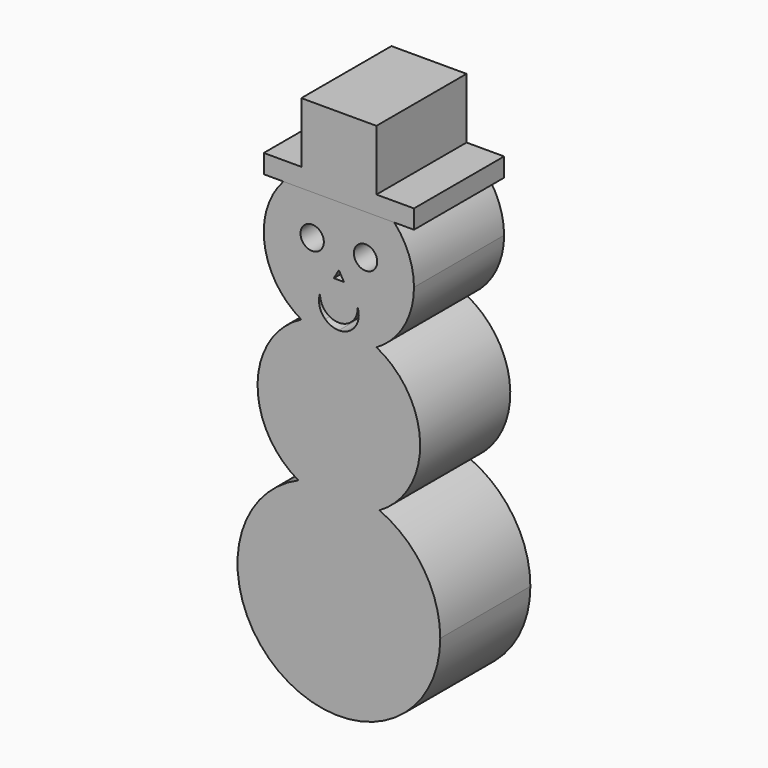
from build123d import *

# Parameters (mm, degrees)
F0_R     = 3.9452510547
F1_DEPTH = 38.1
F2_W     = 12.7
F2_H     = 20.4561264838
F3_DEPTH = 38.1
F4_DEPTH = 38.1


with BuildPart() as f1:
    # F0 (on Front) → F1 (new body)
    with BuildSketch(Plane.XZ):
        with BuildLine():
            ThreePointArc((13.7157117337, -23.8302700758), (23.8025510421, -13.7637598111), (27.4955, 0))
            ThreePointArc((27.4955, 0), (23.5116729393, 14.2549554838), (12.714626341, 24.3791057518))
            ThreePointArc((12.714626341, 24.3791057518), (0, 20.9677), (-12.714626341, 24.3791057518))
            ThreePointArc((-12.714626341, 24.3791057518), (-27.4895738801, 0.5708310965), (-13.7157117337, -23.8302700758))
            ThreePointArc((-13.7157117337, -23.8302700758), (0, -20.9677), (13.7157117337, -23.8302700758))
        make_face()
        with BuildLine():
            ThreePointArc((-12.714626341, 24.3791057518), (0, 20.9677), (12.714626341, 24.3791057518))
            ThreePointArc((12.714626341, 24.3791057518), (8.7732416217, 26.0582568814), (4.6188620822, 27.1047714123))
            ThreePointArc((4.6188620822, 27.1047714123), (2.4852773653, 25.7442761783), (0, 25.2683271861))
            ThreePointArc((0, 25.2683271861), (-2.4852773653, 25.7442761783), (-4.6188620822, 27.1047714123))
            ThreePointArc((-4.6188620822, 27.1047714123), (-8.7732416217, 26.0582568814), (-12.714626341, 24.3791057518))
        make_face()
        with BuildLine():
            ThreePointArc((4.6188620822, 27.1047714123), (8.7732416217, 26.0582568814), (12.714626341, 24.3791057518))
            ThreePointArc((12.714626341, 24.3791057518), (22.0012671119, 33.6750152773), (25.4, 46.3677))
            ThreePointArc((25.4, 46.3677), (-12.6926847227, 68.3689671119), (-12.714626341, 24.3791057518))
            ThreePointArc((-12.714626341, 24.3791057518), (-8.7732416217, 26.0582568814), (-4.6188620822, 27.1047714123))
            ThreePointArc((-4.6188620822, 27.1047714123), (-6.538891729, 30.4166180357), (-6.3411390434, 34.2396712366))
            ThreePointArc((-6.3411390434, 34.2396712366), (-4.6071647855, 29.5343692183), (0, 27.5543271861))
            ThreePointArc((0, 27.5543271861), (4.6071647855, 29.5343692183), (6.3411390434, 34.2396712366))
            ThreePointArc((6.3411390434, 34.2396712366), (6.538891729, 30.4166180357), (4.6188620822, 27.1047714123))
        make_face()
        with Locations((-9.0252510547, 49.9191674486)):
            Circle(F0_R, mode=Mode.SUBTRACT)
        Polygon((-1.7050582101, 40.2543271861), (0, 43.2075746357), (1.7050582101, 40.2543271861), align=None, mode=Mode.SUBTRACT)
        with Locations((9.0252510547, 49.9191674486)):
            Circle(F0_R, mode=Mode.SUBTRACT)
        with BuildLine():
            ThreePointArc((34.29, -55.2577), (28.6889861737, -36.4761619287), (13.7157117337, -23.8302700758))
            ThreePointArc((13.7157117337, -23.8302700758), (0, -27.4955), (-13.7157117337, -23.8302700758))
            ThreePointArc((-13.7157117337, -23.8302700758), (-18.7815380713, -83.9466861737), (34.29, -55.2577))
        make_face()
        with BuildLine():
            ThreePointArc((-13.7157117337, -23.8302700758), (0, -27.4955), (13.7157117337, -23.8302700758))
            ThreePointArc((13.7157117337, -23.8302700758), (0, -20.9677), (-13.7157117337, -23.8302700758))
        make_face()
    extrude(amount=F1_DEPTH)

    # F2 (on Front) → F4 (join)
    with BuildSketch(Plane.XZ):
        with Locations((6.35, 80.0780632419)):
            Rectangle(F2_W, F2_H)
        Polygon((12.7, 69.85), (0, 69.85), (0, 63.5), (25.4, 63.5), (25.4, 69.85), align=None)
        with Locations((-6.35, 80.0780632419)):
            Rectangle(F2_W, F2_H)
        Polygon((0, 63.5), (0, 69.85), (-12.7, 69.85), (-25.4, 69.85), (-25.4, 63.5), align=None)
    extrude(amount=F4_DEPTH)


with BuildPart() as f3:
    # F2 (on Front) → F3 (new body)
    with BuildSketch(Plane.XZ):
        with Locations((6.35, 80.0780632419)):
            Rectangle(F2_W, F2_H)
        Polygon((12.7, 69.85), (0, 69.85), (0, 63.5), (25.4, 63.5), (25.4, 69.85), align=None)
        with Locations((-6.35, 80.0780632419)):
            Rectangle(F2_W, F2_H)
        Polygon((0, 63.5), (0, 69.85), (-12.7, 69.85), (-25.4, 69.85), (-25.4, 63.5), align=None)
    extrude(amount=F3_DEPTH)


solid = Compound([f1.part, f3.part])
